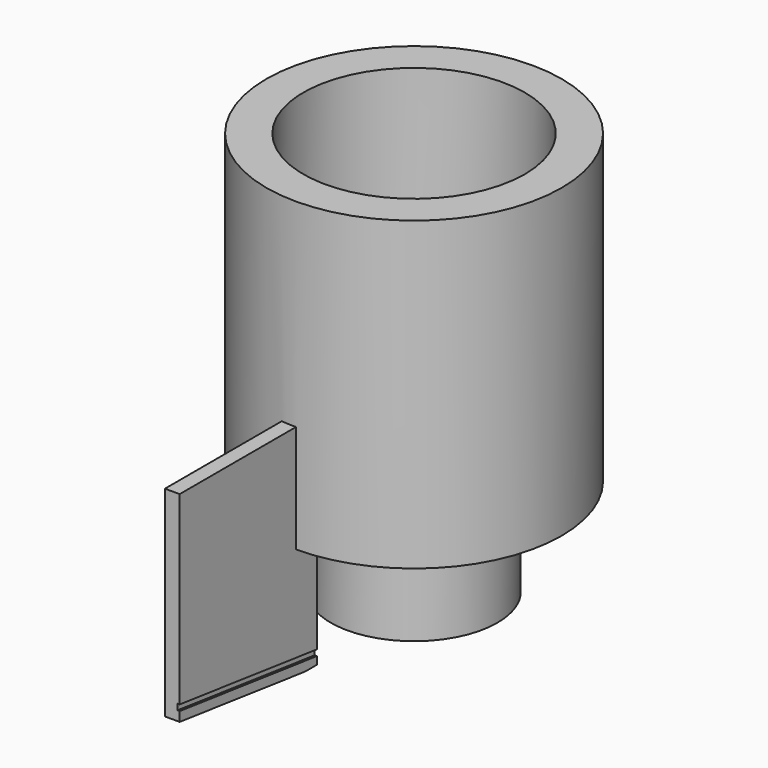
from build123d import *

# Parameters (mm, degrees)
F0_R     = 10
F0_R_2   = 5.65
F1_DEPTH = 2
F2_R     = 10
F2_R_2   = 7
F3_DEPTH = 10.75
F4_R     = 10
F4_R_2   = 7.5
F5_DEPTH = 8
F6_DEPTH = 6.6
F8_DEPTH = 1
F9_DEPTH = 0.15


# Not quite as in the source:
# - a feature names something its author has since deleted; it is built from what else it names


with BuildPart() as f1:
    # F0 (on Top) → F1 (new body)
    with BuildSketch(Plane.XY):
        Circle(F0_R)
        Circle(F0_R_2, mode=Mode.SUBTRACT)
    extrude(amount=F1_DEPTH)

    # F2 (on face) → F3 (join)
    with BuildSketch(Plane.XY.offset(2)):
        Circle(F2_R)
        Circle(F2_R_2, mode=Mode.SUBTRACT)
    extrude(amount=F3_DEPTH)

    # F4 (on face) → F5 (join)
    with BuildSketch(Plane.XY.offset(12.75)):
        Circle(F4_R)
        Circle(F4_R_2, mode=Mode.SUBTRACT)
    extrude(amount=F5_DEPTH)

    # F7 (on Right) → F8 (join)
    with BuildSketch(Plane.YZ):
        Polygon((-19.8482480398, -5.2409250216), (-8.2270988125, -6.6807134215), (-8.2270988125, 1.9598644681), (-8.2270988125, 7.3028788902), (-19.8482480398, 7.3028788902), align=None)
        Polygon((-9.2270988125, -7.6), (-8.2270988125, -7.6), (-8.2270988125, -7.0807134215), (-19.8482480398, -5.6409250216), (-19.8482480398, -6.2841054055), align=None)
        Polygon((-19.8482480398, -5.4409250216), (-8.2270988125, -6.8807134215), (-8.2270988125, -6.6807134215), (-19.8482480398, -5.2409250216), align=None)
        Polygon((-19.8482480398, -5.6409250216), (-8.2270988125, -7.0807134215), (-8.2270988125, -6.8807134215), (-19.8482480398, -5.4409250216), align=None)
    extrude(amount=-F8_DEPTH)

    # F7 (on Right) → F9 (cut)
    with BuildSketch(Plane.YZ):
        Polygon((-19.8482480398, -5.4409250216), (-8.2270988125, -6.8807134215), (-8.2270988125, -6.6807134215), (-19.8482480398, -5.2409250216), align=None)
        Polygon((-19.8482480398, -5.6409250216), (-8.2270988125, -7.0807134215), (-8.2270988125, -6.8807134215), (-19.8482480398, -5.4409250216), align=None)
    extrude(amount=-F9_DEPTH, mode=Mode.SUBTRACT)


with BuildPart() as f6:
    # F0 (on Top) → F6 (new body)
    with BuildSketch(Plane.XY):
        Circle(F0_R_2)
    extrude(amount=-F6_DEPTH)


solid = Compound([f1.part, f6.part])
